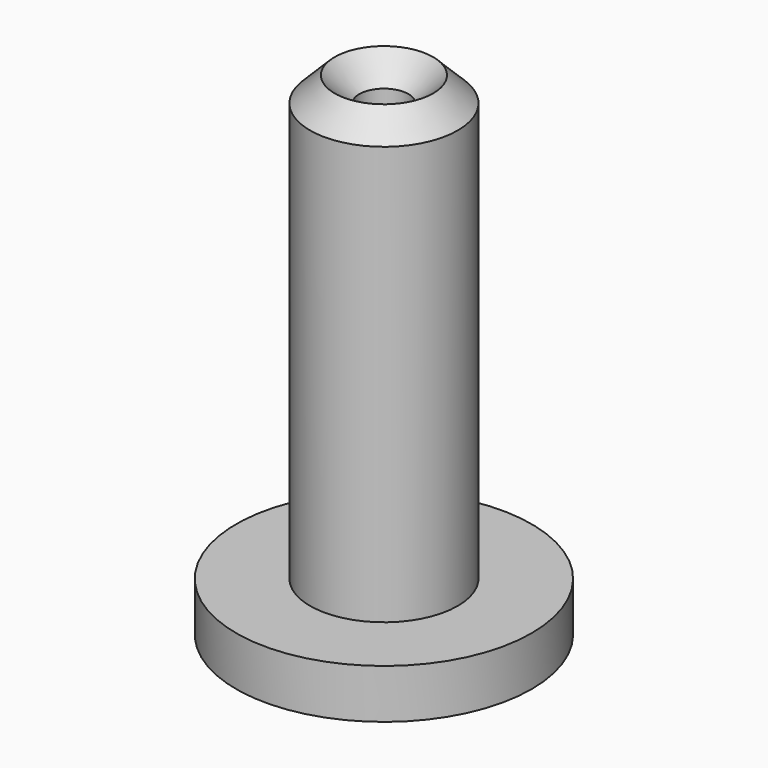
from build123d import *

# Parameters (mm, degrees)
F0_R     = 6
F0_R_2   = 2
F1_DEPTH = 40
F0_R_3   = 12
F2_DEPTH = 4
F3_SIZE  = 1.99999


# Not quite as in the source:
# - a fillet or chamfer is up to 0.001 mm smaller than in the source, because OpenCascade refuses the exact size


with BuildPart() as f1:
    # F0 (on Top) → F1 (new body)
    with BuildSketch(Plane.XY):
        Circle(F0_R)
        Circle(F0_R_2, mode=Mode.SUBTRACT)
    extrude(amount=F1_DEPTH)

    # F0 (on Top) → F2 (join)
    with BuildSketch(Plane.XY):
        Circle(F0_R_3)
        Circle(F0_R, mode=Mode.SUBTRACT)
    extrude(amount=F2_DEPTH)

    # F3 (size 2 in the source; OpenCascade refuses exactly that, so slightly less here)
    f3_edges = [f1.edges().sort_by_distance(p)[0] for p in [
        (-6, 0, 40),
        (-2, 0, 40),
        (-2, 0, 0),
    ]]
    chamfer(f3_edges, length=F3_SIZE)


solid = f1.part
